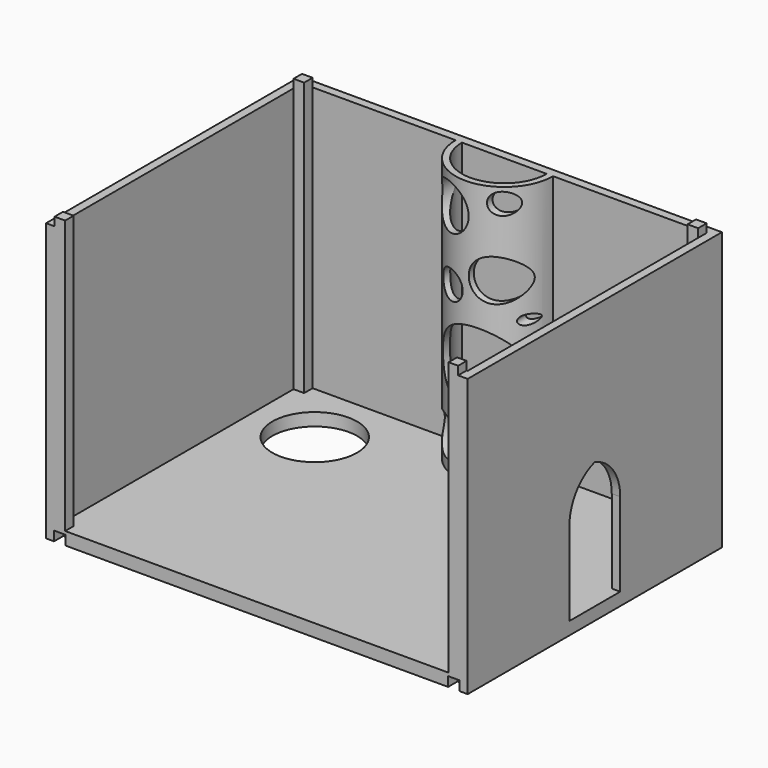
from build123d import *

# Parameters (mm, degrees)
F0_W      = 5
F0_H      = 5
F1_DEPTH  = 125
F2_DEPTH  = 6
F3_W      = 5
F3_H      = 5
F3_W_2    = 4.5
F4_DEPTH  = 4
F5_W      = 5.5
F5_H      = 5.5
F6_DEPTH  = 4.5
F5_R      = 20
F7_DEPTH  = 25
F9_DEPTH  = 25
F10_R     = 10.5485016942
F10_R_2   = 5.0535829712
F10_R_3   = 9.8754590545
F10_R_4   = 17.8823064921
F10_R_5   = 6.6595132661
F10_R_6   = 2.2824643728
F10_R_7   = 8.9411528958
F10_R_8   = 4.3120053672
F11_DEPTH = 97.8


with BuildPart() as f1:
    # F0 (on Top) → F1 (new body)
    with BuildSketch(Plane.XY):
        with BuildLine():
            Line((97.9463080764, 94.0890025382), (-101.0536919236, 94.0890025382))
            Line((-101.0536919236, 94.0890025382), (-101.0536919236, -55.9109974618))
            Line((-101.0536919236, -55.9109974618), (-97.0536919236, -55.9109974618))
            Line((-97.0536919236, -55.9109974618), (-97.0536919236, -50.9109974618))
            Line((-97.0536919236, -50.9109974618), (-97.0536919236, 85.0890025382))
            Line((-97.0536919236, 85.0890025382), (-97.0536919236, 90.0890025382))
            Line((-97.0536919236, 90.0890025382), (-92.0536919236, 90.0890025382))
            Line((-92.0536919236, 90.0890025382), (-24.5536919236, 90.0890025382))
            ThreePointArc((-24.5536919236, 90.0890025382), (-1.5536919236, 67.0890025382), (21.4463080764, 90.0890025382))
            Line((21.4463080764, 90.0890025382), (88.9463080764, 90.0890025382))
            Line((88.9463080764, 90.0890025382), (93.9463080764, 90.0890025382))
            Line((93.9463080764, 90.0890025382), (93.9463080764, 85.0890025382))
            Line((93.9463080764, 85.0890025382), (93.9463080764, -50.9109974618))
            Line((93.9463080764, -50.9109974618), (93.9463080764, -55.9109974618))
            Line((93.9463080764, -55.9109974618), (97.9463080764, -55.9109974618))
            Line((97.9463080764, -55.9109974618), (97.9463080764, 94.0890025382))
        make_face()
        with BuildLine():
            ThreePointArc((18.4463080764, 90.0890025382), (-1.5536919236, 70.0890025382), (-21.5536919236, 90.0890025382))
            Line((-21.5536919236, 90.0890025382), (18.4463080764, 90.0890025382))
        make_face(mode=Mode.SUBTRACT)
        with Locations((-94.5536919236, -53.4109974618)):
            Rectangle(F0_W, F0_H)
        with Locations((91.4463080764, -53.4109974618)):
            Rectangle(F0_W, F0_H)
        with Locations((91.4463080764, 87.5890025382)):
            Rectangle(F0_W, F0_H)
        with Locations((-94.5536919236, 87.5890025382)):
            Rectangle(F0_W, F0_H)
    extrude(amount=F1_DEPTH)

    # F0 (on Top) → F2 (join)
    with BuildSketch(Plane.XY):
        with BuildLine():
            Line((97.9463080764, 94.0890025382), (-101.0536919236, 94.0890025382))
            Line((-101.0536919236, 94.0890025382), (-101.0536919236, -55.9109974618))
            Line((-101.0536919236, -55.9109974618), (-97.0536919236, -55.9109974618))
            Line((-97.0536919236, -55.9109974618), (-97.0536919236, -50.9109974618))
            Line((-97.0536919236, -50.9109974618), (-97.0536919236, 85.0890025382))
            Line((-97.0536919236, 85.0890025382), (-97.0536919236, 90.0890025382))
            Line((-97.0536919236, 90.0890025382), (-92.0536919236, 90.0890025382))
            Line((-92.0536919236, 90.0890025382), (-24.5536919236, 90.0890025382))
            ThreePointArc((-24.5536919236, 90.0890025382), (-1.5536919236, 67.0890025382), (21.4463080764, 90.0890025382))
            Line((21.4463080764, 90.0890025382), (88.9463080764, 90.0890025382))
            Line((88.9463080764, 90.0890025382), (93.9463080764, 90.0890025382))
            Line((93.9463080764, 90.0890025382), (93.9463080764, 85.0890025382))
            Line((93.9463080764, 85.0890025382), (93.9463080764, -50.9109974618))
            Line((93.9463080764, -50.9109974618), (93.9463080764, -55.9109974618))
            Line((93.9463080764, -55.9109974618), (97.9463080764, -55.9109974618))
            Line((97.9463080764, -55.9109974618), (97.9463080764, 94.0890025382))
        make_face()
        with BuildLine():
            ThreePointArc((18.4463080764, 90.0890025382), (-1.5536919236, 70.0890025382), (-21.5536919236, 90.0890025382))
            Line((-21.5536919236, 90.0890025382), (18.4463080764, 90.0890025382))
        make_face(mode=Mode.SUBTRACT)
        with Locations((91.4463080764, -53.4109974618)):
            Rectangle(F0_W, F0_H)
        with Locations((-94.5536919236, -53.4109974618)):
            Rectangle(F0_W, F0_H)
        with Locations((-94.5536919236, 87.5890025382)):
            Rectangle(F0_W, F0_H)
        with Locations((91.4463080764, 87.5890025382)):
            Rectangle(F0_W, F0_H)
        with BuildLine():
            Line((-92.0536919236, -50.9109974618), (-92.0536919236, -55.9109974618))
            Line((-92.0536919236, -55.9109974618), (88.9463080764, -55.9109974618))
            Line((88.9463080764, -55.9109974618), (88.9463080764, -50.9109974618))
            Line((88.9463080764, -50.9109974618), (93.9463080764, -50.9109974618))
            Line((93.9463080764, -50.9109974618), (93.9463080764, 85.0890025382))
            Line((93.9463080764, 85.0890025382), (88.9463080764, 85.0890025382))
            Line((88.9463080764, 85.0890025382), (88.9463080764, 90.0890025382))
            Line((88.9463080764, 90.0890025382), (21.4463080764, 90.0890025382))
            ThreePointArc((21.4463080764, 90.0890025382), (-1.5536919236, 67.0890025382), (-24.5536919236, 90.0890025382))
            Line((-24.5536919236, 90.0890025382), (-92.0536919236, 90.0890025382))
            Line((-92.0536919236, 90.0890025382), (-92.0536919236, 85.0890025382))
            Line((-92.0536919236, 85.0890025382), (-97.0536919236, 85.0890025382))
            Line((-97.0536919236, 85.0890025382), (-97.0536919236, -50.9109974618))
            Line((-97.0536919236, -50.9109974618), (-92.0536919236, -50.9109974618))
        make_face()
    extrude(amount=-F2_DEPTH)

    # F3 (on face) → F4 (join)
    with BuildSketch(Plane.XY.offset(125)):
        with Locations((-94.5536919236, 87.5890025382)):
            Rectangle(F3_W, F3_H)
        with Locations((91.1963080764, -53.4109974618)):
            Rectangle(F3_W_2, F3_H)
        with Locations((91.4463080764, 87.5890025382)):
            Rectangle(F3_W, F3_H)
        with Locations((-94.5536919236, -53.4109974618)):
            Rectangle(F3_W, F3_H)
    extrude(amount=F4_DEPTH)

    # F5 (on face) → F6 (cut)
    with BuildSketch(Plane(origin=(0, 0, -6), x_dir=(1, 0, 0), z_dir=(0, 0, -1))):
        with Locations((-94.5536919236, 53.1609974618)):
            Rectangle(F5_W, F5_H)
        with Locations((-94.5536919236, -87.5890025382)):
            Rectangle(F5_W, F5_H)
        with Locations((91.4463080764, 53.1609974618)):
            Rectangle(F5_W, F5_H)
        with Locations((91.4463080764, -87.5890025382)):
            Rectangle(F5_W, F5_H)
    extrude(amount=-F6_DEPTH, mode=Mode.SUBTRACT)

    # F5 (on face) → F7 (cut)
    with BuildSketch(Plane(origin=(0, 0, -6), x_dir=(1, 0, 0), z_dir=(0, 0, -1))):
        with Locations((-67.0536919236, -60.0890025382)):
            Circle(F5_R)
    extrude(amount=-F7_DEPTH, mode=Mode.SUBTRACT)

    # F8 (on face) → F9 (cut)
    with BuildSketch(Plane.YZ.offset(97.9463080764)):
        with BuildLine():
            Line((4.0890025382, 39.4580720926), (4.0890025382, 0))
            Line((4.0890025382, 0), (19.0890025382, 0))
            Line((19.0890025382, 0), (19.0890025382, 60))
            ThreePointArc((19.0890025382, 60), (8.2381396963, 52.1758824599), (4.0890025382, 39.4580720926))
        make_face()
        with BuildLine():
            Line((19.0890025382, 60), (19.0890025382, 0))
            Line((19.0890025382, 0), (34.0890025382, 0))
            Line((34.0890025382, 0), (34.0890025382, 39.4580720926))
            ThreePointArc((34.0890025382, 39.4580720926), (29.9398653801, 52.1758824599), (19.0890025382, 60))
        make_face()
    extrude(amount=-F9_DEPTH, mode=Mode.SUBTRACT)

    # F10 (on face) → F11 (cut)
    with BuildSketch(Plane.XZ.offset(-90.0890025382)):
        with Locations((-10.5643654242, 110.7224822044)):
            Circle(F10_R)
        with Locations((12.2985364869, 117.9848089814)):
            Circle(F10_R_2)
        with Locations((9.877759032, 85.9767496586)):
            Circle(F10_R_3)
        with Locations((1.2705510017, 47.5132800639)):
            Circle(F10_R_4)
        with Locations((-9.4884643331, 78.714415431)):
            Circle(F10_R_5)
        with Locations((18.4463080764, 69.0313056111)):
            Circle(F10_R_6)
        with Locations((-14.0610439703, 13.8913644478)):
            Circle(F10_R_7)
        with Locations((8.2639073953, 14.429314062)):
            Circle(F10_R_8)
    extrude(amount=F11_DEPTH, mode=Mode.SUBTRACT)


solid = f1.part
